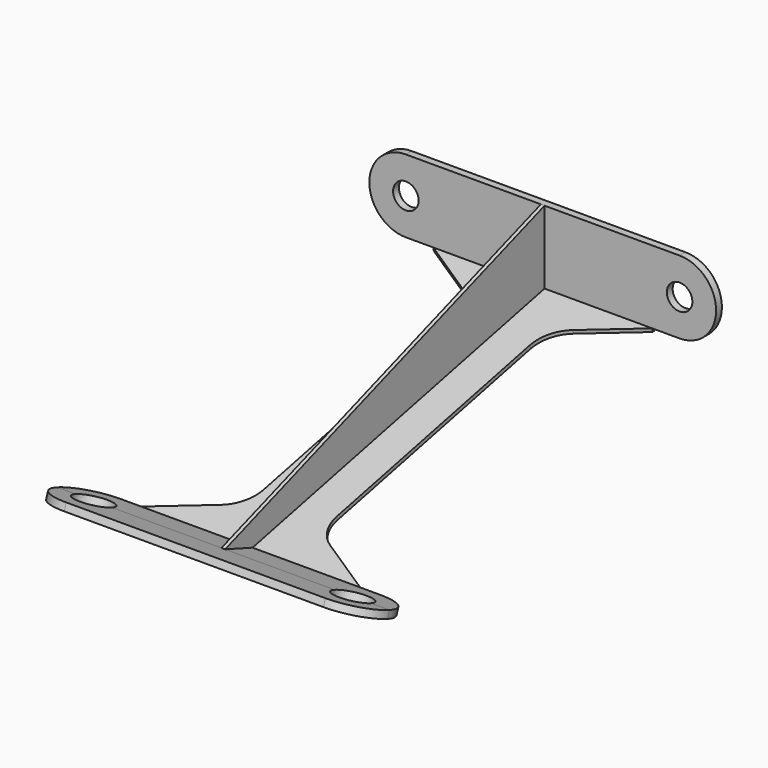
from build123d import *

# Parameters (mm, degrees)
F0_R      = 3.5
F1_DEPTH  = 2
F3_DEPTH  = 0.5
F4_DEPTH  = 45.5
F5_R      = 9.99999
F7_D      = 10
F9_DEPTH  = 30
F11_DEPTH = 23.6012824615
F12_R     = 10


# Not quite as in the source:
# - a fillet or chamfer is up to 0.001 mm smaller than in the source, because OpenCascade refuses the exact size
# - a pattern or mirror of a feature is missing from the dataset's text; its kind, count and spacing are read off the source's solid


with BuildPart() as f1:
    # F0 (on Front) → F1 (new body)
    with BuildSketch(Plane.XZ):
        with BuildLine():
            Line((37.5, 10), (-37.5, 10))
            ThreePointArc((-37.5, 10), (-47.5, 0), (-37.5, -10))
            Line((-37.5, -10), (37.5, -10))
            ThreePointArc((37.5, -10), (47.5, 0), (37.5, 10))
        make_face()
        with Locations((-37.5, 0)):
            Circle(F0_R, mode=Mode.SUBTRACT)
        with Locations((37.5, 0)):
            Circle(F0_R, mode=Mode.SUBTRACT)
    extrude(amount=F1_DEPTH)


with BuildPart() as f3:
    # F2 (on Right) → F3 (new body, symmetric)
    with BuildSketch(Plane.YZ):
        Polygon((-111.3969262079, -28.4202014333), (-102, -31.8404028665), (-2, -10), (-2, 10), align=None)
    extrude(amount=F3_DEPTH, both=True)


with BuildPart() as f4:
    # F2 (on Right) → F4 (new body, symmetric)
    with BuildSketch(Plane.YZ):
        Polygon((-102.6840402867, -33.7197881081), (-102, -31.8404028665), (-111.3969262079, -28.4202014333), (-120.7938524157, -25), (-121.4778927024, -26.8793852416), align=None)
    extrude(amount=F4_DEPTH, both=True)

    # F5 (radius 10 in the source; OpenCascade refuses exactly that, so slightly less here)
    f5_edges = [f4.edges().sort_by_distance(p)[0] for p in [
        (45.5, -121.135873, -25.939693),
        (45.5, -102.34202, -32.780095),
        (-45.5, -121.135873, -25.939693),
        (-45.5, -102.34202, -32.780095),
    ]]
    fillet(f5_edges, radius=F5_R)

    # F7 (through all)
    with Locations(Plane(origin=(0, -22.8490819126, -62.7773366101), x_dir=(1, 0, 0), z_dir=(0, -0.3420201433, -0.9396926208))):
        with Locations((35.5, 94.9585881682), (-35.5, 94.9585881682)):
            Hole(F7_D / 2)


with BuildPart() as f9:
    # F8 (on Right) → F9 (new body, symmetric)
    with BuildSketch(Plane.YZ):
        Polygon((-2, -10), (-102, -31.8404028665), (-102.4047222734, -32.952368174), (0, -10.5867642751), (0, -10), align=None)
    extrude(amount=F9_DEPTH, both=True)

    # F10 (on face) → F11 (cut, through all)
    with BuildSketch(Plane(origin=(0, 1.9935468262, -9.1277932845), x_dir=(1, 0, 0), z_dir=(0, -0.2133742988, 0.976970526))):
        Polygon((30, -106.4449172836), (30, -4.0876840396), (10, -15.6346894234), (10, -94.8979118998), align=None)
    f11 = extrude(amount=-F11_DEPTH, mode=Mode.SUBTRACT)

    # F11_copies: F11 across plane
    add(f11.mirror(Plane(origin=(0, 0, 0), x_dir=(0, 0, -1), z_dir=(-1, 0, 0))), mode=Mode.SUBTRACT)

    # F12
    f12_edges = [f9.edges().sort_by_distance(p)[0] for p in [
        (10, -90.612229, -29.865054),
        (10, -13.174397, -12.952319),
        (-10, -13.174397, -12.952319),
        (-10, -90.612229, -29.865054),
    ]]
    fillet(f12_edges, radius=F12_R)


solid = Compound([f1.part, f3.part, f4.part, f9.part])
